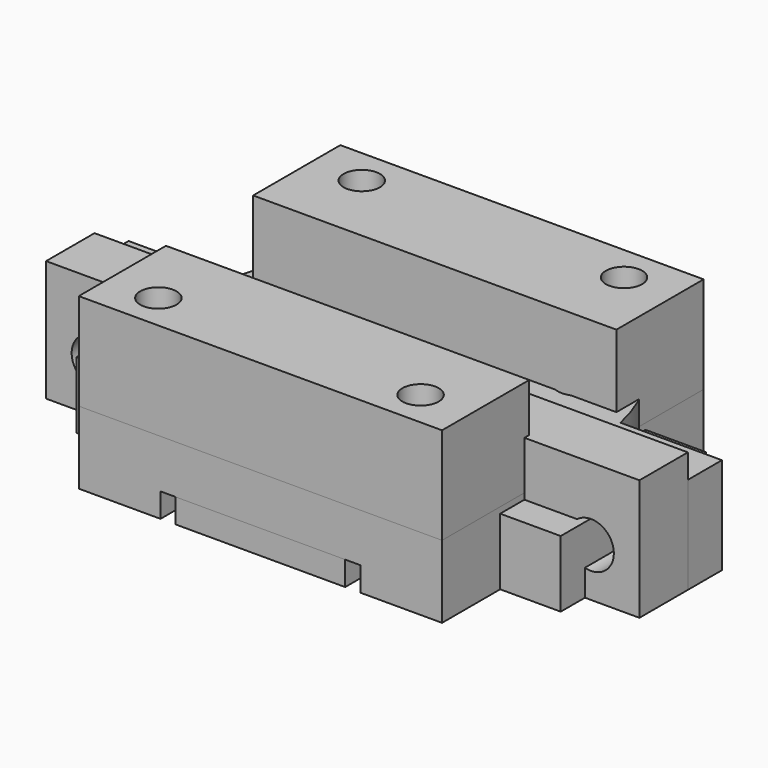
from build123d import *

# Parameters (mm, degrees)
F0_R      = 1.5
F0_W      = 30
F0_H      = 6
F1_DEPTH  = 14
F3_DEPTH  = 8.5
F4_R      = 1.5
F5_DEPTH  = 6
F6_W      = 16.5
F6_H      = 27
F7_DEPTH  = 2
F8_W      = 8
F8_H      = 6
F9_DEPTH  = 5
F10_R     = 1.75
F11_DEPTH = 8
F12_R     = 1.75
F13_DEPTH = 25
F14_W     = 49
F14_H     = 5
F15_DEPTH = 10
F16_R     = 1.8877590654
F17_DEPTH = 8


with BuildPart() as f1:
    # F0 (on Top) → F1 (new body)
    with BuildSketch(Plane.XY):
        Polygon((-15, 7.5), (-20, 7.5), (-20, -7.5), (-15, -7.5), (15, -7.5), (20, -7.5), (20, 7.5), (15, 7.5), align=None)
        with Locations((-16, 0)):
            Circle(F0_R, mode=Mode.SUBTRACT)
        with Locations((16, 0)):
            Circle(F0_R, mode=Mode.SUBTRACT)
        with Locations((0, 10.5)):
            Rectangle(F0_W, F0_H)
        with Locations((-10.828246883, 10.5)):
            Circle(F0_R, mode=Mode.SUBTRACT)
        with Locations((10.828246883, 10.5)):
            Circle(F0_R, mode=Mode.SUBTRACT)
        with Locations((0, -10.5)):
            Rectangle(F0_W, F0_H)
        with Locations((-10.828246883, -10.5)):
            Circle(F0_R, mode=Mode.SUBTRACT)
        with Locations((10.828246883, -10.5)):
            Circle(F0_R, mode=Mode.SUBTRACT)
    extrude(amount=F1_DEPTH)

    # F2 (on face) → F3 (cut)
    with BuildSketch(Plane.XY.offset(14)):
        Polygon((15, 4.5), (-15, 4.5), (-15, 7.5), (-20, 7.5), (-20, 4.5), (-20, -4.5), (-20, -7.5), (-15, -7.5), (-15, -4.5), (15, -4.5), (15, -7.5), (20, -7.5), (20, -4.5), (20, 4.5), (20, 7.5), (15, 7.5), align=None)
    extrude(amount=-F3_DEPTH, mode=Mode.SUBTRACT)

    # F8 (on face) → F9 (cut)
    with BuildSketch(Plane(origin=(0, 0, 0), x_dir=(1, 0, 0), z_dir=(0, 0, -1))):
        with Locations((-11, 10.5)):
            Rectangle(F8_W, F8_H)
        with Locations((11, 10.5)):
            Rectangle(F8_W, F8_H)
        with Locations((-11, -10.5)):
            Rectangle(F8_W, F8_H)
        with Locations((11, -10.5)):
            Rectangle(F8_W, F8_H)
    extrude(amount=-F9_DEPTH, mode=Mode.SUBTRACT)


with BuildPart() as f5:
    # F4 (on Top) → F5 (new body)
    with BuildSketch(Plane.XY):
        Polygon((15, 13.5), (-15, 13.5), (-15, 4.5), (-9.5, 4.5), (-9.5, -4.5), (-15, -4.5), (-15, -13.5), (15, -13.5), (15, -4.5), (9.5, -4.5), (9.5, 4.5), (15, 4.5), align=None)
        with Locations((-10.828246883, -10.5)):
            Circle(F4_R, mode=Mode.SUBTRACT)
        with Locations((10.828246883, -10.5)):
            Circle(F4_R, mode=Mode.SUBTRACT)
        with Locations((-10.828246883, 10.5)):
            Circle(F4_R, mode=Mode.SUBTRACT)
        with Locations((10.828246883, 10.5)):
            Circle(F4_R, mode=Mode.SUBTRACT)
    extrude(amount=F5_DEPTH)

    # F6 (on face) → F7 (cut)
    with BuildSketch(Plane(origin=(0, 0, 0), x_dir=(1, 0, 0), z_dir=(0, 0, -1))):
        Rectangle(F6_W, F6_H)
    extrude(amount=-F7_DEPTH, mode=Mode.SUBTRACT)


with BuildPart() as f11:
    # F10 (on Top) → F11 (new body)
    with BuildSketch(Plane.XY):
        with BuildLine():
            Line((-24.5, 0), (-16.5, 0))
            Line((-16.5, 0), (-8.25, 0))
            Line((-8.25, 0), (-8.25, 2))
            Line((-8.25, 2), (8.25, 2))
            Line((8.25, 2), (8.25, 0))
            Line((8.25, 0), (16.5, 0))
            Line((16.5, 0), (24.5, 0))
            Line((24.5, 0), (24.5, 3.5153171048))
            Line((24.5, 3.5153171048), (16.1211831344, 3.5153171048))
            ThreePointArc((16.1211831344, 3.5153171048), (0, 16.5), (-16.1211831344, 3.5153171048))
            Line((-16.1211831344, 3.5153171048), (-24.5, 3.5153171048))
            Line((-24.5, 3.5153171048), (-24.5, 0))
        make_face()
        with Locations((-10.6088111964, 6.125)):
            Circle(F10_R, mode=Mode.SUBTRACT)
        with Locations((10.6088111964, 6.125)):
            Circle(F10_R, mode=Mode.SUBTRACT)
        with Locations((0, 12.25)):
            Circle(F10_R, mode=Mode.SUBTRACT)
    extrude(amount=F11_DEPTH)

    # F12 (on face) → F13 (cut)
    with BuildSketch(Plane.XZ):
        with Locations((-20.5, 4)):
            Circle(F12_R)
        with Locations((20.5, 4)):
            Circle(F12_R)
    extrude(amount=-F13_DEPTH, mode=Mode.SUBTRACT)


with BuildPart() as f15:
    # F14 (on Top) → F15 (new body)
    with BuildSketch(Plane.XY):
        with Locations((0, -2.5)):
            Rectangle(F14_W, F14_H)
    extrude(amount=F15_DEPTH)

    # F16 (on face) → F17 (cut)
    with BuildSketch(Plane.XZ.offset(5)):
        with Locations((-20.5, 4)):
            Circle(F16_R)
        with Locations((20.5, 4)):
            Circle(F16_R)
    extrude(amount=-F17_DEPTH, mode=Mode.SUBTRACT)


solid = Compound([f1.part, f5.part, f11.part, f15.part])
